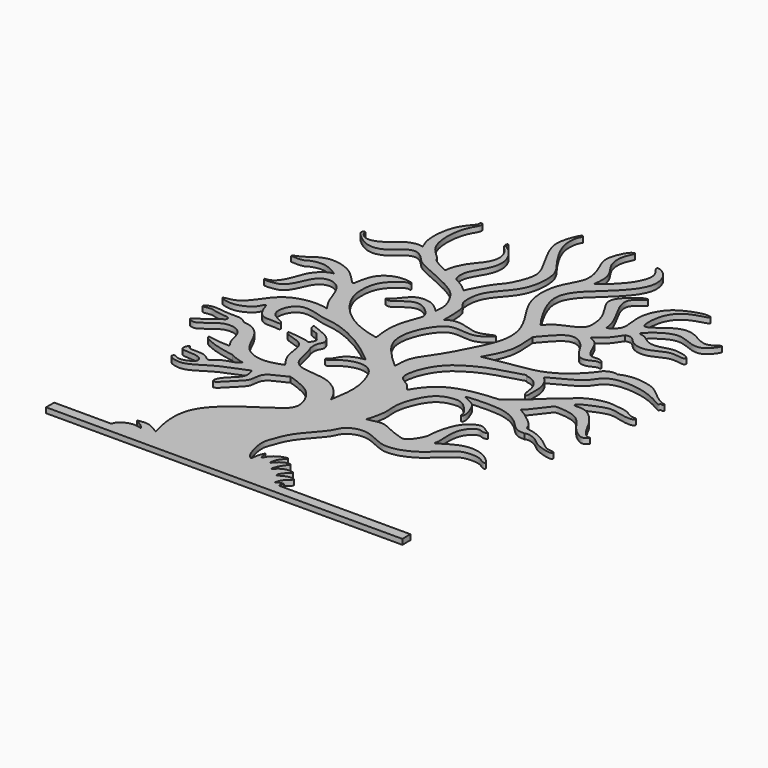
from build123d import *

# Parameters (mm, degrees)
F1_DEPTH = 2.5


with BuildPart() as f1:
    # F0 (on Top) → F1 (new body)
    with BuildSketch(Plane.XY):
        with BuildLine():
            add(Edge.make_bspline(
                [(-37.2274929598, -92.2237484905), (-37.3450221343, -91.7141303732), (-38.1075689973, -88.9113329404), (-43.604203809, -66.4871834906), (-13.8050883231, -50.311066012), (-7.3971472306, -43.5635898817), (-12.2747413738, -32.3520103861), (-19.1758880318, -29.0538192258), (-23.8577212098, -27.2031787778), (-25.7628768968, -26.7645465436)],
                knots=[0, 0, 0, 0, 0.0545700177, 0.1978471329, 0.3800159719, 0.4730400688, 0.5766237722, 0.673699127, 0.7324434095, 0.7324434095, 0.7324434095, 0.7324434095], degree=3))
            add(Edge.make_bspline(
                [(-37.2274929598, -92.2237484905), (-39.0918191693, -91.1772954864), (-42.6840826845, -88.416836232), (-46.4192354741, -89.2437295622), (-48.1499141114, -89.5267036573)],
                knots=[0, 0, 0, 0, 0.5244873249, 1, 1, 1, 1], degree=3))
            add(Edge.make_bspline(
                [(-48.1499141114, -89.5267036573), (-46.6357878306, -90.4674908811), (-44.2239313767, -91.966073771), (-43.5095322249, -93.0738361717), (-43.2436218415, -93.4861624236)],
                knots=[0, 0, 0, 0, 0.6277845758, 1, 1, 1, 1], degree=3))
            add(Edge.make_bspline(
                [(-43.2436218415, -93.4861624236), (-44.8882965758, -93.0891933913), (-48.2154304914, -92.286135435), (-53.3949291569, -95.1532001967), (-53.7720915559, -96.8828718076), (-53.9202807558, -97.5624693836)],
                knots=[0, 0, 0, 0, 0.3724349859, 0.7534262228, 1, 1, 1, 1], degree=3))
            Line((-53.9202807558, -97.5624693836), (-81.071741879, -97.5624693836))
            Line((-81.071741879, -97.5624693836), (-81.071741879, -102.3542508483))
            Line((-81.071741879, -102.3542508483), (87.7496376634, -102.3542508483))
            Line((87.7496376634, -102.3542508483), (87.7496376634, -97.5624693836))
            Line((87.7496376634, -97.5624693836), (25.3826770931, -97.5624693836))
            add(Edge.make_bspline(
                [(2.7441565001, -86.2271991735), (3.0649576654, -86.4877621622), (3.9226400012, -87.1843938983), (3.7489579396, -84.0626662774), (5.7107236383, -79.7859768356), (5.5231648482, -81.4206726001), (6.4364191587, -85.8311109103), (7.4902559788, -80.0930787062), (16.8578873722, -77.0416564355), (11.65799249, -81.2015150502), (10.8430692164, -87.002339468), (13.4800479006, -82.0413900173), (19.7985384574, -80.6783225416), (15.753422443, -84.4781538789), (13.9166662126, -90.7660305308), (17.7187709263, -85.0651298777), (25.0027453432, -85.8709500573), (20.4241408494, -88.0940414879), (18.3764148031, -93.0467476205), (22.9297677816, -89.3810300747), (28.4365107044, -89.8345172495), (23.5533501494, -92.5731641837), (22.1303198851, -97.4097204858), (24.0109507829, -95.3342209527), (26.9540697822, -95.069296518), (25.2843145613, -96.8062342989), (25.353745802, -97.3400385756), (25.3826770931, -97.5624693836)],
                knots=[0, 0, 0, 0, 0.0220478557, 0.0589463457, 0.1035639197, 0.1238214863, 0.1624394271, 0.2060103971, 0.2645686368, 0.3092635123, 0.353568852, 0.3966231341, 0.4437756176, 0.4879462626, 0.5345614015, 0.5814356694, 0.6316309126, 0.6725173463, 0.7141269382, 0.7598317223, 0.8026569348, 0.8477738397, 0.8909251521, 0.9199584628, 0.9523041571, 0.9801256278, 1, 1, 1, 1], degree=3))
            add(Edge.make_bspline(
                [(63.4448099184, -5.3100165565), (62.3489798241, -4.026080382), (59.6902493483, -1.5733697237), (52.5246936437, 2.1000011044), (40.9791784126, 1.8442841377), (32.5718486658, 1.3015086843), (40.4121991432, -0.979957722), (42.1644706313, -4.7333719795), (44.1507466926, -9.5403990475), (43.4294603533, -11.9907012519), (42.5007922183, -11.1165665555), (43.3302045469, -10.0558457893), (37.6376496399, -2.646096314), (32.0506958616, -2.6262917013), (24.1614553703, -4.668986663), (19.1537853149, -16.9399166219), (19.0503972183, -22.9539422069), (19.7250585637, -27.2234210065), (17.9045607996, -34.8554988198), (17.0336657263, -36.2656898306), (24.2002426608, -33.6751283255), (28.8838031342, -36.6920542101), (35.7838362593, -39.166194995), (39.3577079303, -40.1259737762), (43.8794505629, -32.4005635432), (43.3390691716, -30.4028156457), (45.6215475695, -16.7556031936), (54.3252556472, -12.1927388855), (57.1672190516, -15.1795606758), (60.3739467176, -16.4544285374), (57.261900737, -17.1565268122), (54.6338125726, -15.3259924395), (49.3917659151, -20.2800443621), (49.0808976319, -28.343835895), (49.6870829232, -32.8864582508), (48.7744509396, -35.4546793762), (51.2692531374, -33.8549781402), (60.2403555323, -28.023598594), (70.3489432727, -31.0224893139), (74.6750300809, -36.0799199187), (72.2155051868, -35.8671678933), (69.8202155609, -33.4729962531), (62.7443864798, -33.3229810043), (58.6684125003, -35.3154595918), (51.4954302008, -42.250250065), (46.2579790718, -46.0557244783), (34.8445781402, -50.0090016029), (24.525848259, -41.9045805331), (14.4863137885, -45.6634487196), (13.2973451957, -51.7383984427), (2.8153962542, -61.4804582011), (0.1297622405, -70.4668990229), (-1.6873704608, -74.4436042147), (0.8024148227, -84.2695220032), (2.2477540273, -85.726722823), (2.7441565001, -86.2271991735)],
                knots=[0.2565098242, 0.2565098242, 0.2565098242, 0.2565098242, 0.2699877012, 0.2866058552, 0.3079609751, 0.3209847766, 0.3342542003, 0.3470621489, 0.3607299006, 0.3685470769, 0.373378434, 0.3791063233, 0.3962135322, 0.4102355084, 0.4264465739, 0.4476202968, 0.4620628183, 0.4748723501, 0.491485421, 0.4961943664, 0.5107188968, 0.5254804354, 0.5414138485, 0.5520471271, 0.568569615, 0.5779595458, 0.599411902, 0.6165376629, 0.6281045801, 0.636894919, 0.6449783993, 0.6550774405, 0.6696182088, 0.6866854587, 0.6997764188, 0.7074432658, 0.7152112982, 0.7345376577, 0.7540821307, 0.7669388194, 0.7732712513, 0.7842594131, 0.7995486755, 0.8125119075, 0.8309095757, 0.846616447, 0.8661919964, 0.8870960253, 0.904645022, 0.9189431326, 0.9413134612, 0.9593051516, 0.9718864346, 0.9903443819, 1, 1, 1, 1], degree=3))
            add(Edge.make_bspline(
                [(70.3299279054, -8.0914211294), (69.8229118638, -8.1161290277), (68.6774838063, -8.1719480111), (66.0619460376, -7.6378394732), (64.36330212, -6.1269733743), (63.4448099184, -5.3100165565)],
                knots=[0, 0, 0, 0, 0.2672659989, 0.6037954401, 1, 1, 1, 1], degree=3))
            add(Edge.make_bspline(
                [(57.1528694622, 5.9377422838), (58.6583740965, 5.0657466), (61.9020131837, 3.1870148983), (67.9182705544, -1.9969888776), (68.0132328204, -4.7044764926), (72.0271311125, -4.8123028517), (79.1618329725, -7.9629793782), (84.1165899869, -13.3229973697), (88.2863448346, -12.6598300641), (88.1302570331, -14.147114945), (86.2188339325, -14.4478908978), (79.2786946384, -12.4680626061), (76.6294598119, -9.2595039077), (72.0238899558, -7.4172183461), (70.4788669352, -7.9277925211), (70.3299279054, -8.0914211294)],
                knots=[0, 0, 0, 0, 0.0142901325, 0.0307883691, 0.0393101485, 0.0500709614, 0.0669901227, 0.0831668426, 0.0937558816, 0.0988530879, 0.106361001, 0.1221271231, 0.1348320646, 0.1477939846, 0.154977762, 0.154977762, 0.154977762, 0.154977762], degree=3))
            add(Edge.make_bspline(
                [(46.0888547819, 7.2681076556), (48.389097888, 8.9711526494), (53.0391503, 12.4139402661), (59.2283106578, 18.9444562111), (65.2248272956, 23.4344221829), (69.3698883004, 28.1272446181), (78.3101889655, 31.0415107636), (84.3492642973, 30.0014055336), (89.1906160219, 29.5230972562), (92.0818101566, 26.7862644392), (95.8301821982, 27.2223761031), (94.5811799808, 24.9914207295), (88.0105430083, 25.8987436476), (82.3368936402, 28.0164413749), (73.424258585, 23.5813727198), (70.709541316, 22.5466154545), (70.1848982241, 20.2919665985), (75.9741269483, 21.8653819143), (82.8340557029, 15.2559244257), (85.5740658138, 9.759402769), (87.1024341968, 7.0397454152), (89.8389629047, 3.8294544983), (91.9012912475, 4.6941422962), (90.2996024527, 3.0945723944), (89.1742834881, 2.4606354871), (87.0322610167, 3.0616332304), (81.9703225746, 6.7596886053), (77.7913079432, 15.4124323593), (66.4987138265, 16.0681887335), (64.8680419451, 15.6719381722), (59.0931540499, 6.9438492604), (57.6204613933, 6.1802054292), (57.1528694622, 5.9377422838)],
                knots=[0, 0, 0, 0, 0.0451402237, 0.0912531399, 0.1328042537, 0.1710476969, 0.2169756267, 0.255219083, 0.2881389744, 0.3187118402, 0.3440129564, 0.3604469845, 0.398296099, 0.4374173288, 0.4846213641, 0.5104426017, 0.5266024041, 0.5587611894, 0.6057138911, 0.6436420889, 0.6714059172, 0.7016746733, 0.7177262709, 0.7361948756, 0.7540854361, 0.7751669242, 0.8126363027, 0.8600627261, 0.9080996446, 0.9289814835, 0.9774510417, 1, 1, 1, 1], degree=3))
            add(Edge.make_bspline(
                [(67.4956362758, 50.3167273957), (69.1916882844, 50.984947455), (73.143455814, 52.5418869352), (84.38951394, 51.1975931661), (89.3377049583, 45.9774898886), (94.8170277294, 42.3307600849), (96.3107845534, 42.6881563043), (96.5258013064, 41.2321336225), (94.4467009736, 41.9736258524), (94.8001220519, 40.5080681689), (92.6137320363, 41.8595530286), (84.7002725098, 46.3198956797), (71.2623178492, 47.731844698), (64.1963989868, 44.4347004502), (62.2518830478, 38.2749168377), (48.1097658634, 32.098111826), (47.8355853375, 31.1388625515), (49.5118596884, 30.0927626182), (52.5641307538, 24.7384674637), (51.758290574, 18.4257268251), (52.3537106048, 16.0658120952), (49.9649282733, 16.0990944296), (50.3407387037, 23.8417590364), (44.8278896628, 28.2336022187), (42.2265294763, 28.0558464488), (41.8001143286, 29.0404980425), (38.9258989904, 27.8611315116), (28.0579198601, 25.1225760256), (22.0851077223, 22.3147237277), (13.1313618692, 17.2365645604), (8.2205686438, 8.7563398988), (6.8644129181, 3.7349731038), (6.1222092606, -2.1113384889), (12.4649815812, -4.3200077718), (14.3241156606, -8.3385690714), (15.1324353279, -6.9359975224), (21.8719043918, 4.700159267), (37.9323460644, 6.9116083555), (46.0888547819, 7.2681076556)],
                knots=[0, 0, 0, 0, 0.0302861271, 0.0707100349, 0.1050345116, 0.1356976222, 0.1488836674, 0.1594880887, 0.1744996582, 0.1846156993, 0.1996853347, 0.2376359581, 0.283668854, 0.3157921017, 0.3478495629, 0.395027852, 0.4037104913, 0.4192679029, 0.4499008489, 0.4817609961, 0.4983680226, 0.5112022081, 0.5437604198, 0.5759488509, 0.5942288651, 0.604118697, 0.6237601175, 0.6654219477, 0.6986637872, 0.7378022604, 0.7761777723, 0.8048841532, 0.8320974017, 0.8631515881, 0.8862591923, 0.8965675425, 0.9386054058, 1, 1, 1, 1], degree=3))
            add(Edge.make_bspline(
                [(61.8416340161, 49.1312120486), (62.9231265501, 49.7393635743), (64.9205296172, 50.8625555376), (66.6860539115, 50.4883291568), (67.4956362758, 50.3167273957)],
                knots=[0, 0, 0, 0, 0.5414493208, 1, 1, 1, 1], degree=3))
            add(Edge.make_bspline(
                [(19.2542266699, 29.7981717948), (21.8919487253, 30.3086236996), (27.2065827844, 31.3371115469), (35.4683619827, 32.5449654839), (48.9142040042, 34.7379655263), (58.813654421, 44.3454125755), (61.8416340161, 49.1312120486)],
                knots=[0, 0, 0, 0, 0.0852328825, 0.1717321123, 0.2821617594, 0.4131476617, 0.4131476617, 0.4131476617, 0.4131476617], degree=3))
            add(Edge.make_bspline(
                [(24.3610660751, 54.0556638357), (24.7870994834, 49.7398355491), (25.6388572533, 41.1113096974), (21.3819220109, 33.5683054765), (19.2542266699, 29.7981717948)],
                knots=[0, 0, 0, 0, 0.500181417, 1, 1, 1, 1], degree=3))
            add(Edge.make_bspline(
                [(41.1572403984, 67.2579470746), (42.7136300839, 66.4744181065), (45.6531196954, 64.994598956), (46.9639318843, 61.2684155728), (49.0608989396, 57.0909743766), (51.2465301629, 54.9167618192), (55.5124641692, 56.1776412838), (57.4967311489, 53.6396133705), (56.2419947447, 53.5337689538), (55.1730943644, 54.0661698319), (50.801994768, 51.256726788), (46.2711417259, 52.8576942077), (43.3539266593, 59.3511004525), (38.7372040702, 63.5771218677), (33.676271766, 63.9573967349), (28.7059245836, 59.2097938512), (25.8243941029, 55.7915507226), (24.3610660751, 54.0556638357)],
                knots=[0, 0, 0, 0, 0.073685517, 0.1391668255, 0.2112726779, 0.266575347, 0.3343404249, 0.3831252543, 0.4103681007, 0.4454051789, 0.5176974171, 0.5863066295, 0.6744883754, 0.7568895505, 0.826872861, 0.9120808208, 1, 1, 1, 1], degree=3))
            add(Edge.make_bspline(
                [(50.2059963262, 76.6134378524), (49.0203270585, 74.6515719999), (46.1297011539, 70.2809214108), (42.61144609, 68.1696673667), (41.1572403984, 67.2579470746)],
                knots=[0.9153661522, 0.9153661522, 0.9153661522, 0.9153661522, 0.9605063334, 1, 1, 1, 1], degree=3))
            add(Edge.make_bspline(
                [(53.8868478917, 81.8279747897), (52.0954612946, 79.928154063), (51.3031833295, 78.4288966603), (50.2059963262, 76.6134378524)],
                knots=[0.8735946215, 0.8735946215, 0.8735946215, 0.8735946215, 0.9153661522, 0.9153661522, 0.9153661522, 0.9153661522], degree=3))
            add(Edge.make_bspline(
                [(41.1572403984, 76.6134378524), (42.6351949795, 77.6894708866), (47.4362168576, 80.0462747024), (43.8659678332, 91.2167783533), (48.2555283991, 100.7261021255), (53.5962346926, 105.3324096143), (63.0791480351, 108.7918143102), (66.2547865159, 107.6679562578), (65.5662736983, 106.6565877536), (58.324588995, 105.3479242588), (52.2759308295, 100.3840862123), (50.1632734072, 93.1123737462), (50.424225147, 83.1236242073), (60.7565211383, 93.8084695131), (68.8346674463, 94.0090767626), (73.936286253, 90.4483985571), (79.2623847733, 88.7435160353), (83.1965155621, 92.5787538899), (84.1240496431, 91.7063147117), (79.7481160268, 85.6668718285), (73.4453760781, 85.7422137723), (64.8277929727, 90.9817190663), (56.4368667929, 84.5323484685), (53.8868478917, 81.8279747897)],
                knots=[0, 0, 0, 0, 0.0400250206, 0.0931757942, 0.1453174653, 0.1899474054, 0.2421578062, 0.2676699832, 0.2799648987, 0.3234457531, 0.3697887528, 0.4167039309, 0.4565236757, 0.5108251565, 0.5576935368, 0.5980836254, 0.6360418462, 0.6715170158, 0.6824067178, 0.7239839444, 0.7645265646, 0.8141333121, 0.8735946215, 0.8735946215, 0.8735946215, 0.8735946215], degree=3))
            add(Edge.make_bspline(
                [(20.759199095, 63.2703550982), (21.875902072, 64.6690030986), (24.4524394441, 67.8960642936), (35.0843064055, 70.8576565453), (35.5936465516, 76.8359775714), (34.1950937507, 84.7197044314), (26.8616712251, 93.1739294181), (30.4925009847, 99.5972251762), (37.6892798676, 105.0487851262), (40.0940569574, 103.622621229), (29.2153725661, 99.240034684), (39.9358405099, 84.3573903337), (40.7946949123, 78.9120585118), (41.1572403984, 76.6134378524)],
                knots=[0, 0, 0, 0, 0.081380759, 0.1877675365, 0.2625673004, 0.3580782832, 0.4648435335, 0.5516378848, 0.6501899265, 0.6819808894, 0.7726036675, 0.9040099071, 1, 1, 1, 1], degree=3))
            add(Edge.make_bspline(
                [(15.5446621577, 101.305804592), (17.2896868094, 102.7211409732), (20.5252387421, 105.3453981127), (23.5901470448, 108.6577650839), (27.4156082502, 113.4384936954), (29.7296573685, 120.9965112979), (25.8348896558, 124.6973241423), (25.6474173526, 126.621485149), (30.9025894426, 124.5722454337), (34.4196292757, 116.8313383065), (30.6504479146, 107.3981213097), (20.0054438799, 97.6471333034), (13.5340167459, 91.6729697087), (9.6782525317, 83.2171492699), (15.3496475288, 70.9679911341), (18.9641410436, 65.5812187906), (20.759199095, 63.2703550982)],
                knots=[0, 0, 0, 0, 0.0679722368, 0.1245420868, 0.1911660594, 0.2638343368, 0.3226841613, 0.3484153459, 0.4033151039, 0.4789888284, 0.5621198352, 0.6640046721, 0.7440065212, 0.8210277546, 0.9171995083, 1, 1, 1, 1], degree=3))
            add(Edge.make_bspline(
                [(-1.0268479206, 4.1595074951), (-0.9804550099, 6.8584952934), (-0.880156747, 12.6905088128), (5.7813551276, 21.0440445549), (12.4079643626, 33.3955682268), (19.3937586535, 48.125130898), (14.9695567272, 62.0149094333), (3.9306787738, 75.5609144988), (4.7017491739, 92.4518357089), (12.4889651932, 101.9442962943), (9.3990392528, 112.1590077395), (5.6163635776, 118.985201345), (8.0489294682, 126.0438511938), (10.3995693062, 129.9756117739), (13.0239860856, 130.3954175575), (9.9174108299, 125.7246148127), (9.8295409015, 117.179286744), (16.5454940896, 110.622864249), (15.8758297422, 104.388023005), (15.5446621577, 101.305804592)],
                knots=[0, 0, 0, 0, 0.0552004248, 0.1171493109, 0.1907808537, 0.2674139715, 0.3389594798, 0.4192846988, 0.495984221, 0.5614500039, 0.6217075332, 0.6752138488, 0.7268981116, 0.768079879, 0.7896413814, 0.8287841717, 0.885104876, 0.9421512597, 1, 1, 1, 1], degree=3))
            add(Edge.make_bspline(
                [(-9.9296377961, 44.185873063), (-9.2466027159, 44.6986388311), (-7.735338022, 45.833170313), (-3.6846383223, 46.3858265511), (1.411372238, 44.9040535925), (6.882290002, 43.2582718213), (11.9509290708, 46.3935066577), (13.8820859844, 46.3114135828), (11.2660735226, 43.6687100653), (5.8306622755, 40.5383004927), (-2.3568475894, 42.47039685), (-7.7750624669, 40.2584469662), (-13.5911870143, 31.0244357094), (-15.5555040819, 17.3731008026), (-6.1998259684, 8.8642528861), (-1.0268479206, 4.1595074951)],
                knots=[0, 0, 0, 0, 0.0506556873, 0.112079385, 0.1842266896, 0.2587234983, 0.3334481645, 0.3637823068, 0.4142743366, 0.4935497707, 0.5816871648, 0.6537281209, 0.7541476934, 0.8640623833, 1, 1, 1, 1], degree=3))
            add(Edge.make_bspline(
                [(-52.6340775449, 85.0807889329), (-53.4417802709, 86.9686157525), (-55.2876001499, 91.2828122502), (-54.4034662485, 102.4663830898), (-50.7936581702, 108.6228837201), (-47.5399061032, 111.8298431865), (-47.9679311794, 112.7458100754), (-47.5912161102, 113.7172615074), (-46.2454310096, 113.1001739902), (-46.6890683043, 110.8926877522), (-48.1824557205, 109.0749984628), (-50.9018956919, 102.1343273273), (-50.7737983853, 91.9608318933), (-47.7988712168, 85.6666600485), (-42.3527620259, 81.4122364508), (-42.2872471878, 79.5691266667), (-36.0141479645, 76.2837841414), (-34.0875356374, 75.5293201915), (-34.5387164976, 77.0876830014), (-31.9928981592, 84.0235897895), (-28.1740348591, 88.0772429446), (-24.7690441513, 93.1328074119), (-24.7852789818, 98.1320343692), (-26.9925910871, 101.9880216303), (-29.2857488794, 103.6353119341), (-29.7615565451, 105.6704178988), (-29.3714767718, 106.7248777471), (-28.1441706237, 105.8565476984), (-29.4163247439, 104.6615950824), (-26.0046192155, 103.3868615416), (-21.3136735601, 96.864512296), (-21.427540894, 89.8880731413), (-24.5841046884, 83.9388794112), (-27.9016166373, 78.7317015616), (-27.486783571, 74.1992257752), (-26.8378622419, 72.2913569145), (-22.899427309, 70.9566796957), (-18.501031884, 66.8248507495), (-19.0160223374, 68.0425371648), (-12.863340998, 79.0435201441), (-9.8103913275, 81.2393827112), (-5.8417469442, 90.1831057754), (-5.495153501, 96.6675760126), (-11.2608232077, 105.9586747105), (-14.8593103904, 113.3406039436), (-16.1172183746, 119.2777771162), (-13.8091023907, 126.543570909), (-11.9977251343, 129.5345622464), (-10.9601345353, 128.1678968719), (-12.1652005986, 127.6074749153), (-13.5258923312, 121.3778215424), (-10.7739176159, 113.4697263104), (-5.3858418421, 105.3386581912), (0.2375059887, 98.5661031078), (-0.7414289749, 85.2135331016), (-5.6151458221, 77.7021486417), (-13.5106113702, 69.8460321036), (-13.7243747662, 58.9234560228), (-9.8065916092, 56.7728819242), (-9.8811595086, 49.1449591548), (-9.9296377961, 44.185873063)],
                knots=[0, 0, 0, 0, 0.0201796955, 0.0461160794, 0.0676540662, 0.0832203262, 0.0902327328, 0.0970168921, 0.1047613206, 0.1155581841, 0.1275650669, 0.1486338938, 0.1737403992, 0.1947609874, 0.2143185126, 0.2246449153, 0.2454024242, 0.2550638896, 0.2626984474, 0.2836378822, 0.3030624942, 0.3219446937, 0.3391225174, 0.3553710887, 0.3684405941, 0.3794118464, 0.3861960562, 0.3937623392, 0.4015600031, 0.4144232671, 0.4365842538, 0.4569793447, 0.4772807441, 0.4968228851, 0.5129250898, 0.5231220451, 0.5396895237, 0.5574554404, 0.5622297811, 0.5893266848, 0.6067135579, 0.630090907, 0.6501497428, 0.6757572221, 0.6984273694, 0.7175598431, 0.739529235, 0.7521460821, 0.7594829724, 0.766869951, 0.7855966388, 0.8087232112, 0.8331483589, 0.8561839323, 0.8837630016, 0.9073931462, 0.9335346906, 0.9576591347, 0.9724732404, 1, 1, 1, 1], degree=3))
            add(Edge.make_bspline(
                [(-16.7333973365, 47.9496394661), (-16.5200707181, 49.8111967442), (-16.0756544434, 53.6893173318), (-19.3364084776, 59.9184207218), (-21.6608688575, 63.1807188258), (-27.4059211182, 67.0920874785), (-38.1241689587, 71.7629088272), (-45.6007705856, 74.9966751167), (-48.2464549171, 78.8599032763), (-52.8290124058, 81.5969934783), (-57.8245577404, 78.6999017771), (-61.57586119, 74.3329979208), (-68.9081647921, 72.5279962388), (-75.1091106554, 76.6917350652), (-78.6332186406, 80.2717891226), (-76.3214739579, 81.6596350844), (-76.8623430727, 79.8255344618), (-72.6271810187, 75.7865860019), (-64.8529805535, 79.6186698263), (-61.1546523749, 84.0911376206), (-55.0250388817, 86.0183504762), (-53.303423498, 85.3432578467), (-52.6340775449, 85.0807889329)],
                knots=[0, 0, 0, 0, 0.0522692542, 0.1088908051, 0.1521866256, 0.2086194524, 0.2847893142, 0.3466005514, 0.3929897323, 0.4400271437, 0.4896405552, 0.5423318142, 0.5992702493, 0.6596987353, 0.703397823, 0.7282118936, 0.7504639926, 0.7978086656, 0.8588773239, 0.9134297681, 0.9663424044, 1, 1, 1, 1], degree=3))
            add(Edge.make_bspline(
                [(-64.7216094412, 47.9496394661), (-66.018222376, 48.7224732338), (-68.655111203, 50.2941656583), (-73.2286145409, 51.7561858889), (-78.5425969811, 50.5156267785), (-80.1417329179, 48.7820995804), (-85.1714465501, 48.9633470775), (-86.2358448119, 48.9852435855), (-85.7716444215, 49.9176194212), (-82.4646063132, 50.7220181307), (-78.7232536888, 54.1169281574), (-72.9433231845, 56.6197998014), (-65.1572501926, 55.0869935403), (-59.5774137236, 51.6402461224), (-54.963355788, 45.9446333075), (-53.9228361319, 46.5365168218), (-53.5995192295, 55.2928862466), (-45.5487587135, 61.6019871789), (-36.8044406539, 60.3340300052), (-37.6739125233, 58.793935896), (-39.1581903935, 60.1242682624), (-48.0599905873, 53.2929347644), (-48.8100192985, 44.5002938416), (-48.4906448362, 38.2092116326), (-42.6639817428, 27.9294375376), (-31.6412001783, 20.0790823464), (-20.680777295, 17.5222140896), (-20.7087940091, 18.270442608), (-22.6663093802, 29.0846638228), (-17.8956030625, 39.4551384819), (-17.3906707709, 42.6364810982), (-19.6132211266, 45.9275740006), (-25.2493913139, 49.8701815596), (-31.0089945982, 46.9867406516), (-34.6136871182, 43.0930002148), (-37.7560383107, 44.0232275515), (-37.1546751118, 44.6974701948), (-35.3438802755, 45.0790277202), (-31.6262633929, 50.8633673058), (-27.4213605003, 53.0984407371), (-21.0190019227, 52.2797040349), (-18.1687210934, 49.3998536469), (-16.7333973365, 47.9496394661)],
                knots=[0, 0, 0, 0, 0.0243344234, 0.0494882995, 0.0751049868, 0.0929102924, 0.1180880036, 0.1279059366, 0.136635461, 0.1569970977, 0.182953744, 0.2111570575, 0.2423963084, 0.273248182, 0.3023830043, 0.3103457791, 0.3419973199, 0.3788697206, 0.4089179963, 0.4179045134, 0.430249896, 0.4660669329, 0.5000254317, 0.5281356993, 0.5660972315, 0.6104722645, 0.6456296617, 0.6510968173, 0.6876327177, 0.727268448, 0.7462726484, 0.7681155971, 0.7967642378, 0.8245927818, 0.850850656, 0.867855798, 0.8752796865, 0.889967959, 0.9193665101, 0.9442985442, 0.9719502647, 1, 1, 1, 1], degree=3))
            add(Edge.make_bspline(
                [(-49.5091502239, 24.4531677211), (-50.6741982972, 26.1900734075), (-53.2564513975, 30.0398116254), (-55.8682083942, 39.9142796437), (-61.674994757, 43.4153407703), (-67.6933473363, 41.8872469106), (-70.3860692014, 34.9672337748), (-73.4351949152, 29.0154452777), (-78.2779270946, 27.9583605892), (-82.401304202, 27.7576574551), (-82.3686074794, 28.7197371549), (-81.8255661392, 28.6568985409), (-78.0089541935, 29.064754793), (-74.4278001225, 36.3030599009), (-72.935896894, 42.4205824318), (-68.1031012193, 47.2197175637), (-65.7214664123, 47.7338123843), (-64.7216094412, 47.9496394661)],
                knots=[0, 0, 0, 0, 0.079660115, 0.1765614516, 0.2519514097, 0.3219988063, 0.4044265478, 0.4820429453, 0.5505035416, 0.6083780668, 0.6287606247, 0.6474223038, 0.702220537, 0.7875203256, 0.8671542078, 0.9442287327, 1, 1, 1, 1], degree=3))
            add(Edge.make_bspline(
                [(-12.5164702042, 1.3666866655), (-16.1367309925, 4.3344742026), (-23.4927229467, 10.3647086308), (-37.3619105698, 17.0008223567), (-45.6685949859, 17.5510553212), (-49.564420068, 18.9046088024), (-58.5184169775, 21.1574218309), (-63.0051590943, 13.8796250086), (-61.9727274426, 7.6463379565), (-55.9512749534, 6.0678352995), (-55.0528042235, 3.7095378317), (-58.6123755522, 4.5881906212), (-65.5027684787, 3.4381772987), (-68.3039827443, 11.7326773823), (-68.5999441447, 12.5858740326), (-69.5223056856, 12.3793805272), (-69.9782715703, 9.2283156934), (-77.884475349, 4.1336453591), (-85.3468108127, 6.5652931139), (-84.7259957504, 7.5853259743), (-77.806486572, 7.6429189623), (-71.9278901812, 17.9069949942), (-65.6071028768, 23.59363506), (-55.7281835352, 25.670904976), (-51.4303657528, 24.8293573324), (-49.5091502239, 24.4531677211)],
                knots=[0, 0, 0, 0, 0.0695023443, 0.1412215074, 0.1922641097, 0.2299735284, 0.2820155937, 0.3311916645, 0.3740066945, 0.4177452862, 0.4387085717, 0.468615247, 0.5154784404, 0.5656719159, 0.5809235447, 0.5944318353, 0.6240544091, 0.6798301083, 0.7265040942, 0.7378631993, 0.7816600551, 0.8438081541, 0.8977277492, 0.9542821389, 1, 1, 1, 1], degree=3))
            add(Edge.make_bspline(
                [(-2.672668481, -31.4833661953), (-1.9495527056, -27.4717327402), (-0.7017982468, -19.7140560763), (-2.9566541704, -10.1949138776), (-6.4241061952, -3.2040038514), (-12.9932836553, -1.6250607901), (-19.941709789, -4.4355315937), (-22.2738035452, -7.438974394), (-24.4955675377, -8.0312649901), (-24.8650586841, -7.0064678291), (-22.9298569516, -6.5633627014), (-21.8416723487, -2.8943437945), (-17.7977051428, 0.4606628846), (-14.2902766298, 1.0623807784), (-12.5164702042, 1.3666866655)],
                knots=[0, 0, 0, 0, 0.1323420234, 0.2517666285, 0.3542964321, 0.4485749422, 0.55142804, 0.6264958207, 0.6776058791, 0.7060126312, 0.7526420368, 0.8254193867, 0.9115900874, 1, 1, 1, 1], degree=3))
            add(Edge.make_bspline(
                [(-34.4120361799, -4.0592065906), (-32.834837884, -6.9770249437), (-32.5156608645, -15.0544084018), (-26.5428272572, -19.576818475), (-14.0789930402, -18.8484994782), (-5.396286275, -25.5395355217), (-3.5038442905, -29.7697320085), (-2.672668481, -31.4833661953)],
                knots=[0.2245803433, 0.2245803433, 0.2245803433, 0.2245803433, 0.3783744283, 0.5164345873, 0.698698358, 0.8684795861, 1, 1, 1, 1], degree=3))
            add(Edge.make_bspline(
                [(-37.9676868369, -0.9149979606), (-37.0038208852, -1.3205765429), (-35.6295858826, -2.1804790046), (-34.7129217829, -3.5025679378), (-34.4120361799, -4.0592065906)],
                knots=[0.1482110562, 0.1482110562, 0.1482110562, 0.1482110562, 0.1952407059, 0.2245803433, 0.2245803433, 0.2245803433, 0.2245803433], degree=3))
            add(Edge.make_bspline(
                [(-48.832975328, 0.8319125627), (-45.2106295124, 0.4101416112), (-41.0052512609, 0.3631580638), (-37.9676868369, -0.9149979606)],
                knots=[0, 0, 0, 0, 0.1482110562, 0.1482110562, 0.1482110562, 0.1482110562], degree=3))
            add(Edge.make_bspline(
                [(-33.2285104425, -20.5735026688), (-34.8126305943, -18.3219866617), (-38.347321489, -13.7620087577), (-37.4795366175, -2.385101079), (-47.9270684971, -1.6187157773), (-48.861077857, 0.5560507904), (-48.832975328, 0.8319125627)],
                knots=[0, 0, 0, 0, 0.2828695608, 0.5827725324, 0.8684913597, 1, 1, 1, 1], degree=3))
            add(Edge.make_bspline(
                [(-66.3896742472, -3.4927321221), (-63.1100361837, -3.4334796618), (-56.408459152, -7.2335453249), (-53.3973839171, -19.8627213445), (-42.1504743291, -23.8706760475), (-35.7096682755, -21.4894980877), (-33.2285104425, -20.5735026688)],
                knots=[0.6000951463, 0.6000951463, 0.6000951463, 0.6000951463, 0.6870170226, 0.8008637914, 0.903876492, 1, 1, 1, 1], degree=3))
            add(Edge.make_bspline(
                [(-73.1798899436, -5.805161018), (-71.6617686125, -4.9010067577), (-69.3287178228, -3.7922302594), (-67.1117308689, -3.5057773516), (-66.3896742472, -3.4927321221)],
                knots=[0.5427921691, 0.5427921691, 0.5427921691, 0.5427921691, 0.5809581211, 0.6000951463, 0.6000951463, 0.6000951463, 0.6000951463], degree=3))
            add(Edge.make_bspline(
                [(-58.7928760131, -21.5203306113), (-59.535264543, -20.4493647491), (-61.5984632606, -17.5905827476), (-62.176702067, -9.4516836967), (-72.747992069, -6.9875017414), (-79.7863132528, -16.2636960514), (-84.7633851473, -13.6425543142), (-81.8519849066, -12.5310191598), (-76.7283000423, -7.9185033721), (-73.1798899436, -5.805161018)],
                knots=[0, 0, 0, 0, 0.0685026022, 0.1544257829, 0.2471153875, 0.3506020809, 0.4064720162, 0.453584247, 0.5427921691, 0.5427921691, 0.5427921691, 0.5427921691], degree=3))
            add(Edge.make_bspline(
                [(-69.5522801538, -20.3152766135), (-67.333267926, -20.7348486768), (-63.2833010809, -21.5006186552), (-60.190916195, -21.5141935293), (-58.7928760131, -21.5203306113)],
                knots=[0, 0, 0, 0, 0.5479087392, 1, 1, 1, 1], degree=3))
            add(Edge.make_bspline(
                [(-53.4929993208, -26.4647400743), (-56.0555222346, -26.0608981956), (-61.83038794, -24.9711712698), (-69.406454912, -21.9566433926), (-69.5262364293, -20.6659277103), (-69.5522801538, -20.3152766135)],
                knots=[0, 0, 0, 0, 0.4377786682, 0.839807764, 1, 1, 1, 1], degree=3))
            add(Edge.make_bspline(
                [(-46.872654434, -28.7683213166), (-49.2496760958, -28.4264399673), (-51.31650374, -27.4674849166), (-53.4929993208, -26.4647400743)],
                knots=[0.924180508, 0.924180508, 0.924180508, 0.924180508, 1, 1, 1, 1], degree=3))
            add(Edge.make_bspline(
                [(-28.4129288048, -26.3526793569), (-29.095885344, -26.2997700168), (-34.2013405009, -26.2129143246), (-41.415694536, -29.1739682068), (-46.1641995491, -28.8702166909), (-46.872654434, -28.7683213166)],
                knots=[0.7587553627, 0.7587553627, 0.7587553627, 0.7587553627, 0.7783885676, 0.9015830322, 0.924180508, 0.924180508, 0.924180508, 0.924180508], degree=3))
            add(Edge.make_bspline(
                [(-25.7628768968, -26.7645465436), (-26.6162087439, -26.5680802615), (-27.4976467362, -26.423587193), (-28.4129288048, -26.3526793569)],
                knots=[0.7324434095, 0.7324434095, 0.7324434095, 0.7324434095, 0.7587553627, 0.7587553627, 0.7587553627, 0.7587553627], degree=3))
        make_face()
        with BuildLine():
            Line((-46.3711405987, -97.5624693836), (-53.9202807558, -97.5624693836))
            add(Edge.make_bspline(
                [(-53.9202807558, -97.5624693836), (-53.024604586, -97.2448206608), (-50.9947674853, -96.5249453482), (-48.0285174117, -97.190560421), (-46.3711405987, -97.5624693836)],
                knots=[0, 0, 0, 0, 0.441255197, 1, 1, 1, 1], degree=3))
        make_face(mode=Mode.SUBTRACT)
        with BuildLine():
            add(Edge.make_bspline(
                [(-28.4129288048, -26.3526793569), (-31.1545593217, -27.1128696018), (-35.7356706428, -29.7218552825), (-39.2178067852, -31.4677990183), (-39.9825319571, -31.8335374413)],
                knots=[0, 0, 0, 0, 0.0782338128, 0.1011718242, 0.1011718242, 0.1011718242, 0.1011718242], degree=3))
            add(Edge.make_bspline(
                [(-28.4129288048, -26.3526793569), (-29.095885344, -26.2997700168), (-34.2013405009, -26.2129143246), (-41.415694536, -29.1739682068), (-46.1641995491, -28.8702166909), (-46.872654434, -28.7683213166)],
                knots=[0.7587553627, 0.7587553627, 0.7587553627, 0.7587553627, 0.7783885676, 0.9015830322, 0.924180508, 0.924180508, 0.924180508, 0.924180508], degree=3))
            add(Edge.make_bspline(
                [(-39.9825319571, -31.8335374413), (-41.4527577478, -32.536689478), (-45.111386699, -34.1072920405), (-52.6712556529, -36.5717527031), (-60.2796601951, -42.1513687679), (-65.8523739779, -43.7887942409), (-71.507637196, -41.5863042751), (-69.7573473205, -39.4742627036), (-67.7515308045, -42.3454813494), (-58.6096245095, -38.7594133643), (-63.3211412032, -33.9526952883), (-73.0720283737, -35.8033938538), (-70.1572808684, -29.6175057137), (-69.6068964071, -33.3671569891), (-61.4334322235, -31.3971916616), (-58.0279957114, -36.6631370916), (-55.2838808472, -31.7539137411), (-47.7312859235, -30.812836129), (-47.2043986727, -29.2198427412), (-46.872654434, -28.7683213166)],
                knots=[0.1011718242, 0.1011718242, 0.1011718242, 0.1011718242, 0.1452714003, 0.2181961944, 0.2933996782, 0.3537320236, 0.4067582983, 0.4336606763, 0.4736162732, 0.5398213514, 0.589588485, 0.6581468857, 0.701240305, 0.7323076959, 0.799171721, 0.8509839152, 0.900412769, 0.9665328729, 1, 1, 1, 1], degree=3))
        make_face()
        with BuildLine():
            add(Edge.make_bspline(
                [(53.8868478917, 81.8279747897), (52.0954612946, 79.928154063), (51.3031833295, 78.4288966603), (50.2059963262, 76.6134378524)],
                knots=[0.8735946215, 0.8735946215, 0.8735946215, 0.8735946215, 0.9153661522, 0.9153661522, 0.9153661522, 0.9153661522], degree=3))
            add(Edge.make_bspline(
                [(50.2059963262, 76.6134378524), (51.2648917141, 76.8175719938), (53.5049474656, 77.2494137756), (55.9841995053, 73.0434942478), (63.9293488976, 71.1990023266), (71.7472398661, 77.4655108969), (78.5719729603, 74.7840792974), (79.9423555241, 77.2567054001), (71.900025761, 79.3639517243), (67.4667917194, 77.3648124384), (60.5646982709, 76.37579145), (56.6866395988, 80.7225025701), (53.1158447932, 80.7860354207), (53.5401512705, 81.2266176047), (53.8868478917, 81.8279747897)],
                knots=[0, 0, 0, 0, 0.0670839925, 0.1474472913, 0.2528484018, 0.3747381525, 0.4719635625, 0.5133125095, 0.6158546447, 0.7079255733, 0.805737355, 0.8989624871, 0.962022402, 1, 1, 1, 1], degree=3))
        make_face()
        with BuildLine():
            add(Edge.make_bspline(
                [(-25.7628768968, -26.7645465436), (-27.5242169642, -27.5650459415), (-30.9089520178, -29.1263080925), (-35.8426946117, -31.9784343078), (-35.2299258245, -38.2464182171), (-39.6043162875, -41.8181367343), (-46.3329469822, -49.5846063), (-46.5308486483, -43.9525470782), (-40.5589421806, -39.2245408529), (-38.7652471107, -35.9806360756), (-39.4615611494, -33.2550257125), (-39.9825319571, -31.8335374413)],
                knots=[0, 0, 0, 0, 0.1172478461, 0.2270137242, 0.3378529302, 0.4594330702, 0.5951734891, 0.6745306782, 0.8102710971, 0.9014831857, 1, 1, 1, 1], degree=3))
            add(Edge.make_bspline(
                [(-25.7628768968, -26.7645465436), (-26.6162087439, -26.5680802615), (-27.4976467362, -26.423587193), (-28.4129288048, -26.3526793569)],
                knots=[0.7324434095, 0.7324434095, 0.7324434095, 0.7324434095, 0.7587553627, 0.7587553627, 0.7587553627, 0.7587553627], degree=3))
            add(Edge.make_bspline(
                [(-28.4129288048, -26.3526793569), (-31.1545593217, -27.1128696018), (-35.7356706428, -29.7218552825), (-39.2178067852, -31.4677990183), (-39.9825319571, -31.8335374413)],
                knots=[0, 0, 0, 0, 0.0782338128, 0.1011718242, 0.1011718242, 0.1011718242, 0.1011718242], degree=3))
        make_face()
        with BuildLine():
            add(Edge.make_bspline(
                [(-34.4120361799, -4.0592065906), (-34.5525081711, -2.5979308067), (-34.8148377009, 0.0816372585), (-32.2814398237, 2.6633903459), (-35.6094844559, 7.3353049516), (-41.2327314572, 9.0418602831), (-44.2147223383, 10.6144300297), (-44.6970543254, 9.9262668708), (-43.4627716134, 6.9664685332), (-39.4962843392, 6.8550086142), (-38.8209260059, 4.2518271231), (-35.4960956321, 2.0793484173), (-37.1066166818, 0.1022161285), (-37.9676868369, -0.9149979606)],
                knots=[0, 0, 0, 0, 0.1038388097, 0.1914433873, 0.3032787174, 0.4335743282, 0.520838794, 0.5545669841, 0.6392306072, 0.7354483219, 0.8156168624, 0.9070757697, 1, 1, 1, 1], degree=3))
            add(Edge.make_bspline(
                [(-37.9676868369, -0.9149979606), (-37.0038208852, -1.3205765429), (-35.6295858826, -2.1804790046), (-34.7129217829, -3.5025679378), (-34.4120361799, -4.0592065906)],
                knots=[0.1482110562, 0.1482110562, 0.1482110562, 0.1482110562, 0.1952407059, 0.2245803433, 0.2245803433, 0.2245803433, 0.2245803433], degree=3))
        make_face()
        with BuildLine():
            add(Edge.make_bspline(
                [(-66.3896742472, -3.4927321221), (-67.3097701246, -2.733981208), (-69.4434360246, -0.9857180731), (-75.8254121207, -1.8089028522), (-83.3222303081, 0.0781564301), (-87.0867837111, -2.2694885621), (-86.0785573546, -3.2613859392), (-82.3671647301, -2.0678649943), (-80.2405551088, -3.4775833298), (-72.2337923197, -3.6491814188), (-72.9601024291, -5.2855384091), (-73.1798899436, -5.805161018)],
                knots=[0, 0, 0, 0, 0.1099539259, 0.2549566831, 0.4197576296, 0.5243839327, 0.5718756325, 0.6791453002, 0.7807432794, 0.9315058961, 1, 1, 1, 1], degree=3))
            add(Edge.make_bspline(
                [(-73.1798899436, -5.805161018), (-71.6617686125, -4.9010067577), (-69.3287178228, -3.7922302594), (-67.1117308689, -3.5057773516), (-66.3896742472, -3.4927321221)],
                knots=[0.5427921691, 0.5427921691, 0.5427921691, 0.5427921691, 0.5809581211, 0.6000951463, 0.6000951463, 0.6000951463, 0.6000951463], degree=3))
        make_face()
        with BuildLine():
            add(Edge.make_bspline(
                [(-53.9202807558, -97.5624693836), (-53.024604586, -97.2448206608), (-50.9947674853, -96.5249453482), (-48.0285174117, -97.190560421), (-46.3711405987, -97.5624693836)],
                knots=[0, 0, 0, 0, 0.441255197, 1, 1, 1, 1], degree=3))
            Line((-53.9202807558, -97.5624693836), (-46.3711405987, -97.5624693836))
        make_face()
    extrude(amount=F1_DEPTH)


solid = f1.part
